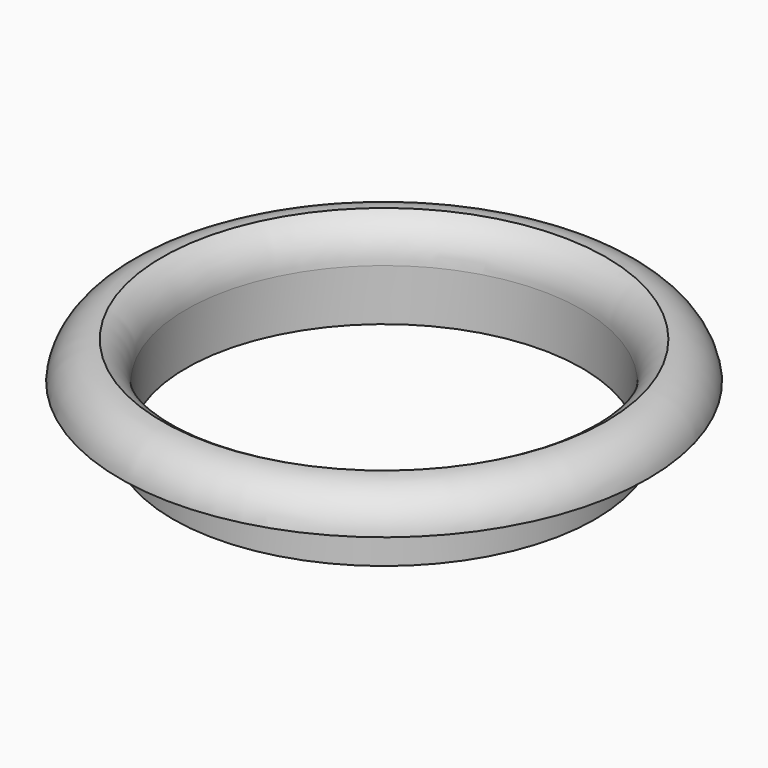
from build123d import *

# Parameters (mm, degrees)
F0_R     = 25.4
F0_R_2   = 23.8125
F1_DEPTH = 6.35
F0_R_3   = 31.75
F2_DEPTH = 4.445
F5_DEPTH = 3.175


# Not quite as in the source:
# - a fillet or chamfer that OpenCascade refuses, or shapes differently, is made with other operations: its cross-section is extruded or revolved along the edge and cut away or added


with BuildPart() as f1:
    # F0 (on Top) → F1 (new body)
    with BuildSketch(Plane.XY):
        Circle(F0_R)
        Circle(F0_R_2, mode=Mode.SUBTRACT)
    extrude(amount=-F1_DEPTH)

    # F0 (on Top) → F2 (join)
    with BuildSketch(Plane.XY):
        Circle(F0_R_3)
        Circle(F0_R, mode=Mode.SUBTRACT)
        Circle(F0_R)
        Circle(F0_R_2, mode=Mode.SUBTRACT)
    extrude(amount=F2_DEPTH)

    # F3: fillet of radius 5.08 on 1 edges, made by hand

    # F3_s1 → F3_t2 (revolve, cut)
    with BuildSketch(Plane.XZ):
        with BuildLine():
            ThreePointArc((31.75, 0), (30.0699479175, 3.175), (26.7098437524, 4.445))
            Line((26.7098437524, 4.445), (31.75, 4.445))
            Line((31.75, 4.445), (31.75, 0))
        make_face()
    revolve(axis=Axis((0, 0, 4.445), (0, 0, 1)), mode=Mode.SUBTRACT)

    # F4: fillet of radius 5.08 on 1 edges, made by hand

    # F4_s1 → F4_t2 (revolve, cut)
    with BuildSketch(Plane.XZ):
        with BuildLine():
            ThreePointArc((26.7098437524, 4.445), (24.5974858127, 2.5705934827), (23.8125, -0.1422008573))
            Line((23.8125, -0.1422008573), (23.8125, 4.445))
            Line((23.8125, 4.445), (26.7098437524, 4.445))
        make_face()
    revolve(axis=Axis((0, 0, 4.445), (0, 0, 1)), mode=Mode.SUBTRACT)


with BuildPart() as f5:
    # F0 (on Top) → F5 (new body)
    with BuildSketch(Plane.XY):
        Circle(F0_R_3)
        Circle(F0_R, mode=Mode.SUBTRACT)
    extrude(amount=F5_DEPTH)

    # F6: fillet of radius 5.08 on 1 edges, made by hand

    # F6_s1 → F6_t2 (revolve, cut)
    with BuildSketch(Plane.XZ):
        with BuildLine():
            ThreePointArc((31.75, 0), (29.8805202921, 2.3071134838), (27.0407139607, 3.175))
            Line((27.0407139607, 3.175), (31.75, 3.175))
            Line((31.75, 3.175), (31.75, 0))
        make_face()
    revolve(axis=Axis((0, 0, 3.175), (0, 0, 1)), mode=Mode.SUBTRACT)


solid = Compound([f1.part, f5.part])
